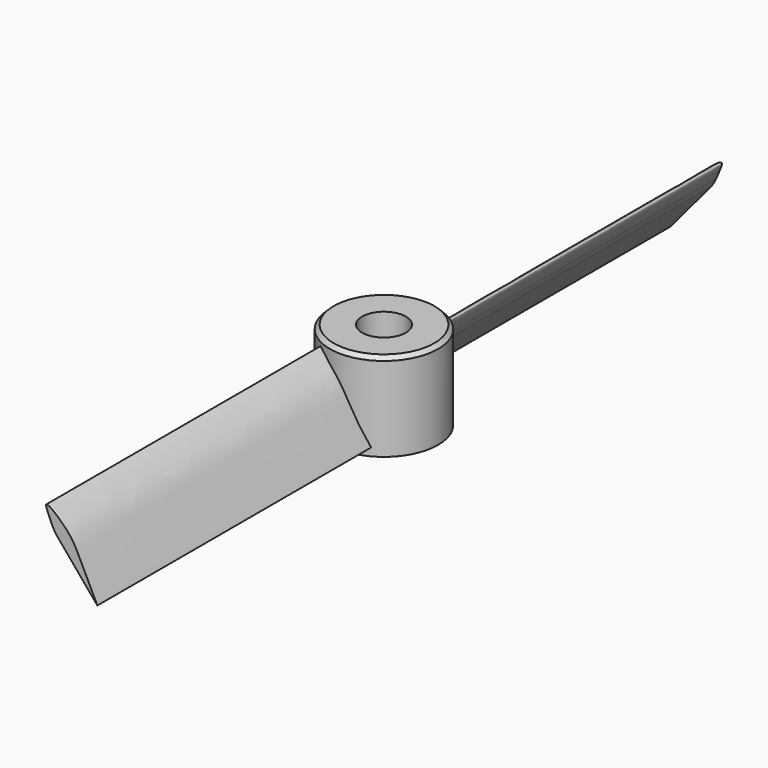
from build123d import *

# Parameters (mm, degrees)
F0_R     = 7.05
F0_R_2   = 2.85
F1_DEPTH = 11.5
F3_DEPTH = 50.8
F4_R     = 5
F6_DEPTH = 50.8
F7_R     = 5
F8_SIZE  = 0.5
F9_DEPTH = 25


# Not quite as in the source:
# - a feature names something its author has since deleted; it is built from what else it names


with BuildPart() as f1:
    # F0 (on Top) → F1 (new body)
    with BuildSketch(Plane.XY):
        Circle(F0_R)
        Circle(F0_R_2, mode=Mode.SUBTRACT)
        Circle(F0_R_2)
    extrude(amount=F1_DEPTH)

    # F2 (on Front) → F3 (join)
    with BuildSketch(Plane.XZ):
        with BuildLine():
            add(Edge.make_bspline(
                [(-2.3585223883, 7.7854411997), (-2.8747237345, 9.1404017243), (-4.2513498132, 11.5661629184), (-0.7257173445, 8.6840933061), (0.5291966234, 6.8089567189), (1.9158112194, 3.812674118), (2.8421595437, 1.9518426304), (3.3105071745, 1.0221040932)],
                knots=[0, 0, 0, 0, 0.1977876363, 0.3919769243, 0.5835513721, 0.7917756861, 1, 1, 1, 1], degree=3))
            Line((-2.3585223883, 7.7854411997), (3.3105071745, 1.0221040932))
        make_face()
    extrude(amount=F3_DEPTH)

    # F4
    f4_edges = [f1.edges().sort_by_distance(p)[0] for p in [
        (-2.358522, -28.721892, 7.785441),
    ]]
    fillet(f4_edges, radius=F4_R)

    # F5 (on Front) → F6 (join)
    with BuildSketch(Plane.XZ):
        with BuildLine():
            Line((-3.3105030617, 1.0221070312), (2.3585265011, 7.7854441377))
            add(Edge.make_bspline(
                [(2.3585265011, 7.7854441377), (2.8747278473, 9.1404046623), (4.251353926, 11.5661658564), (0.7257214573, 8.6840962441), (-0.5291925106, 6.8089596569), (-1.9158071066, 3.812677056), (-2.8421554309, 1.9518455683), (-3.3105030617, 1.0221070312)],
                knots=[0, 0, 0, 0, 0.1977876363, 0.3919769243, 0.5835513721, 0.7917756861, 1, 1, 1, 1], degree=3))
        make_face()
    extrude(amount=-F6_DEPTH)

    # F7
    f7_edges = [f1.edges().sort_by_distance(p)[0] for p in [
        (2.358527, 28.721892, 7.785444),
    ]]
    fillet(f7_edges, radius=F7_R)

    # F8
    f8_edges = [f1.edges().sort_by_distance(p)[0] for p in [
        (-7.05, 0, 11.5),
    ]]
    chamfer(f8_edges, length=F8_SIZE)

    # F0 (on Top) → F9 (cut)
    with BuildSketch(Plane.XY):
        Circle(F0_R_2)
    extrude(amount=F9_DEPTH, mode=Mode.SUBTRACT)


solid = f1.part
